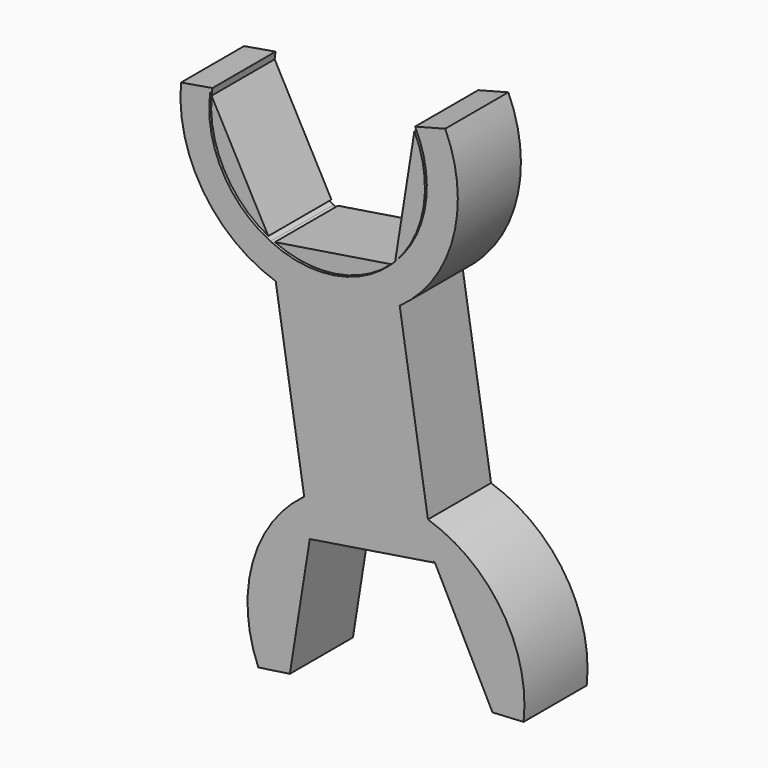
from build123d import *

# Parameters (mm, degrees)
F1_DEPTH = 12.7


with BuildPart() as f1:
    # F0 (on Front) → F1 (new body)
    with BuildSketch(Plane.XZ):
        with BuildLine():
            Line((-48.7995083992, -1.5905502483), (-28.8532047719, 1.556229154))
            Line((-28.8532047719, 1.556229154), (-28.8777340522, 1.7117114456))
            ThreePointArc((-28.8777340522, 1.7117114456), (-39.3680005528, 3.2542025696), (-48.7995083992, -1.5905502483))
        make_face()
        with BuildLine():
            ThreePointArc((-48.7995083992, -1.5905502483), (-39.3680005528, 3.2542025696), (-28.8777340522, 1.7117114456))
            Line((-28.8777340522, 1.7117114456), (-29.7704133367, 7.3700845868))
            ThreePointArc((-29.7704133367, 7.3700845868), (-40.124753878, 8.1269858394), (-49.6992845111, 4.1128071308))
            Line((-49.6992845111, 4.1128071308), (-48.7995083992, -1.5905502483))
        make_face()
        with BuildLine():
            Line((-29.7704133367, 7.3700845868), (-28.8777340522, 1.7117114456))
            ThreePointArc((-28.8777340522, 1.7117114456), (-28.7564587611, 1.6516025926), (-28.6356556912, 1.5905502483))
            ThreePointArc((-28.6356556912, 1.5905502483), (-21.0516796779, -6.0026344403), (-19.3792761761, -16.6033991491))
            Line((-19.3792761761, -16.6033991491), (-14.3672252335, -16.3208022891))
            ThreePointArc((-14.3672252335, -16.3208022891), (-17.8363108802, -1.7234938217), (-29.7704133367, 7.3700845868))
        make_face()
        with BuildLine():
            ThreePointArc((-52.0050752019, -21.7505278741), (-53.6774787037, -11.1497631653), (-48.7995083992, -1.5905502483))
            Line((-48.7995083992, -1.5905502483), (-49.6992845111, 4.1128071308))
            ThreePointArc((-49.6992845111, 4.1128071308), (-58.0095489431, -7.9058060898), (-57.0933466821, -22.4889515699))
            Line((-57.0933466821, -22.4889515699), (-52.0050752019, -21.7505278741))
        make_face()
        with BuildLine():
            Line((-52.0050752019, -21.7505278741), (-48.7995083992, -1.5905502483))
            ThreePointArc((-48.7995083992, -1.5905502483), (-53.6774787037, -11.1497631653), (-52.0050752019, -21.7505278741))
        make_face()
        with BuildLine():
            ThreePointArc((-19.3792761761, -16.6033991491), (-21.0516796779, -6.0026344403), (-28.6356556912, 1.5905502483))
            Line((-28.6356556912, 1.5905502483), (-19.3792761761, -16.6033991491))
        make_face()
        with BuildLine():
            ThreePointArc((-49.6992845111, 4.1128071308), (-40.124753878, 8.1269858394), (-29.7704133367, 7.3700845868))
            Line((-29.7704133367, 7.3700845868), (-34.3175456617, 36.1927220814))
            ThreePointArc((-34.3175456617, 36.1927220814), (-43.9369802174, 32.2901614466), (-54.2815496204, 33.1581387178))
            Line((-54.2815496204, 33.1581387178), (-49.6992845111, 4.1128071308))
        make_face()
        with BuildLine():
            ThreePointArc((-54.2815496204, 33.1581387178), (-43.9369802174, 32.2901614466), (-34.3175456617, 36.1927220814))
            Line((-34.3175456617, 36.1927220814), (-35.1863457074, 41.6997333097))
            Line((-35.1863457074, 41.6997333097), (-35.6492351188, 41.6267067032))
            ThreePointArc((-35.6492351188, 41.6267067032), (-44.912324279, 37.0560431574), (-55.1326493347, 38.5529539073))
            Line((-55.1326493347, 38.5529539073), (-54.2815496204, 33.1581387178))
        make_face()
        with BuildLine():
            Line((-35.1863457074, 41.6997333097), (-34.3175456617, 36.1927220814))
            ThreePointArc((-34.3175456617, 36.1927220814), (-25.7156020352, 48.6101817009), (-26.9856018058, 63.6625515522))
            Line((-26.9856018058, 63.6625515522), (-31.8412224938, 62.388399532))
            ThreePointArc((-31.8412224938, 62.388399532), (-30.168818992, 51.7876348232), (-35.0467892965, 42.2284219061))
            ThreePointArc((-35.0467892965, 42.2284219061), (-35.3443246218, 41.9238722412), (-35.6492351188, 41.6267067032))
            Line((-35.6492351188, 41.6267067032), (-35.1863457074, 41.6997333097))
        make_face()
        with BuildLine():
            ThreePointArc((-69.5354928411, 56.3773410221), (-65.958395671, 42.107159461), (-54.2815496204, 33.1581387178))
            Line((-54.2815496204, 33.1581387178), (-55.1326493347, 38.5529539073))
            ThreePointArc((-55.1326493347, 38.5529539073), (-62.9027913452, 45.9601983724), (-64.8350992238, 56.5199599082))
            Line((-64.8350992238, 56.5199599082), (-64.6096867091, 56.1025407975))
            ThreePointArc((-64.6096867091, 56.1025407975), (-64.5477640968, 56.6730847269), (-64.4670215196, 57.241270807))
            Line((-64.4670215196, 57.241270807), (-69.5354928411, 56.3773410221))
        make_face()
    extrude(amount=F1_DEPTH)


with BuildPart() as f1b:
    # F0 (on Front) → F1, piece 2 (new body)
    with BuildSketch(Plane.XZ):
        with BuildLine():
            Line((-35.6869321752, 41.62075952), (-54.4145137861, 38.6662487912))
            ThreePointArc((-54.4145137861, 38.6662487912), (-44.611914547, 37.3620552095), (-35.6869321752, 41.62075952))
        make_face()
    extrude(amount=F1_DEPTH)


with BuildPart() as f1c:
    # F0 (on Front) → F1, piece 3 (new body)
    with BuildSketch(Plane.XZ):
        with BuildLine():
            ThreePointArc((-64.6096867091, 56.1025407975), (-62.5969769393, 46.2635354492), (-55.473616533, 39.1843572918))
            Line((-55.473616533, 39.1843572918), (-64.6096867091, 56.1025407975))
        make_face()
    extrude(amount=F1_DEPTH)


with BuildPart() as f1d:
    # F0 (on Front) → F1, piece 4 (new body)
    with BuildSketch(Plane.XZ):
        with BuildLine():
            Line((-31.9493958213, 61.7080918062), (-35.0467892965, 42.2284219061))
            ThreePointArc((-35.0467892965, 42.2284219061), (-30.4648884431, 51.4859577882), (-31.9493958213, 61.7080918062))
        make_face()
    extrude(amount=F1_DEPTH)


solid = Compound([f1.part, f1b.part, f1c.part, f1d.part])
